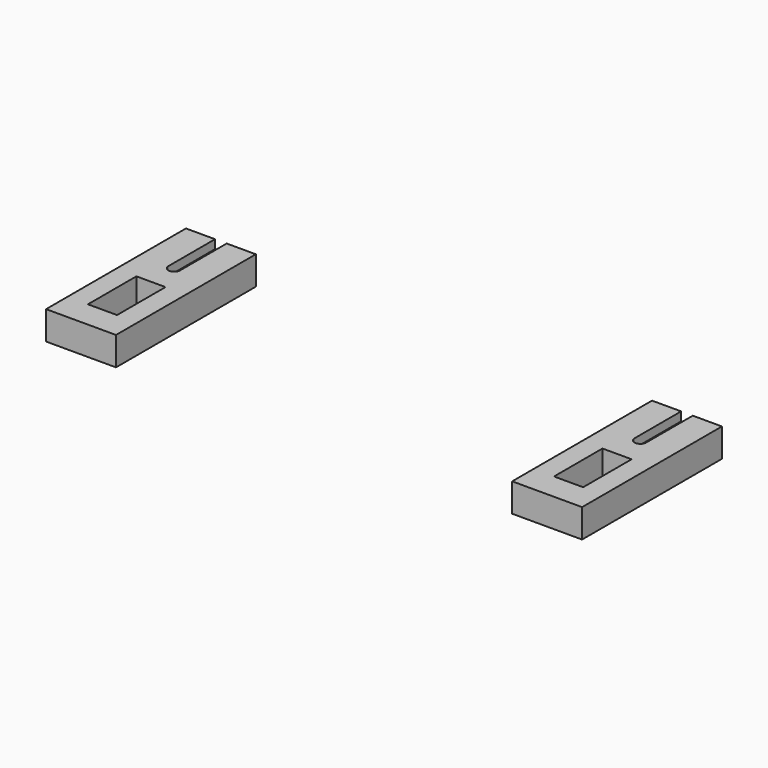
from build123d import *

# Parameters (mm, degrees)
F0_W     = 6.35
F0_H     = 13.208
F1_DEPTH = 6.223
F2_DEPTH = 4.318


with BuildPart() as f1:
    # F0 (on Top) → F1 (new body)
    with BuildSketch(Plane.XY):
        with BuildLine():
            Line((43.18, -12.7), (58.42, -12.7))
            Line((58.42, -12.7), (58.42, 25.4))
            Line((58.42, 25.4), (52.07, 25.4))
            Line((52.07, 25.4), (52.07, 12.7))
            ThreePointArc((52.07, 12.7), (50.8, 11.43), (49.53, 12.7))
            Line((49.53, 12.7), (49.53, 25.4))
            Line((49.53, 25.4), (43.18, 25.4))
            Line((43.18, 25.4), (43.18, -12.7))
        make_face()
        with Locations((50.8, -0.254)):
            Rectangle(F0_W, F0_H, mode=Mode.SUBTRACT)
    extrude(amount=F1_DEPTH)

    # F0 (on Top) → F2 (join)
    with BuildSketch(Plane.XY):
        with BuildLine():
            Line((52.07, 12.7), (52.07, 25.4))
            Line((52.07, 25.4), (49.53, 25.4))
            Line((49.53, 25.4), (49.53, 12.7))
            ThreePointArc((49.53, 12.7), (50.8, 13.97), (52.07, 12.7))
        make_face()
    extrude(amount=F2_DEPTH)


with BuildPart() as f1b:
    # F0 (on Top) → F1, piece 2 (new body)
    with BuildSketch(Plane.XY):
        with BuildLine():
            Line((-58.42, 25.4), (-58.42, -12.7))
            Line((-58.42, -12.7), (-43.18, -12.7))
            Line((-43.18, -12.7), (-43.18, 25.4))
            Line((-43.18, 25.4), (-49.53, 25.4))
            Line((-49.53, 25.4), (-49.53, 12.7))
            ThreePointArc((-49.53, 12.7), (-50.8, 11.43), (-52.07, 12.7))
            Line((-52.07, 12.7), (-52.07, 25.4))
            Line((-52.07, 25.4), (-58.42, 25.4))
        make_face()
        with Locations((-50.8, -0.254)):
            Rectangle(F0_W, F0_H, mode=Mode.SUBTRACT)
    extrude(amount=F1_DEPTH)


with BuildPart() as f2:
    # F0 (on Top) → F2, piece 2 (new body)
    with BuildSketch(Plane.XY):
        with BuildLine():
            Line((-49.53, 25.4), (-52.07, 25.4))
            Line((-52.07, 25.4), (-52.07, 12.7))
            ThreePointArc((-52.07, 12.7), (-50.8, 13.97), (-49.53, 12.7))
            Line((-49.53, 12.7), (-49.53, 25.4))
        make_face()
    extrude(amount=F2_DEPTH)


solid = Compound([f1.part, f1b.part, f2.part])
